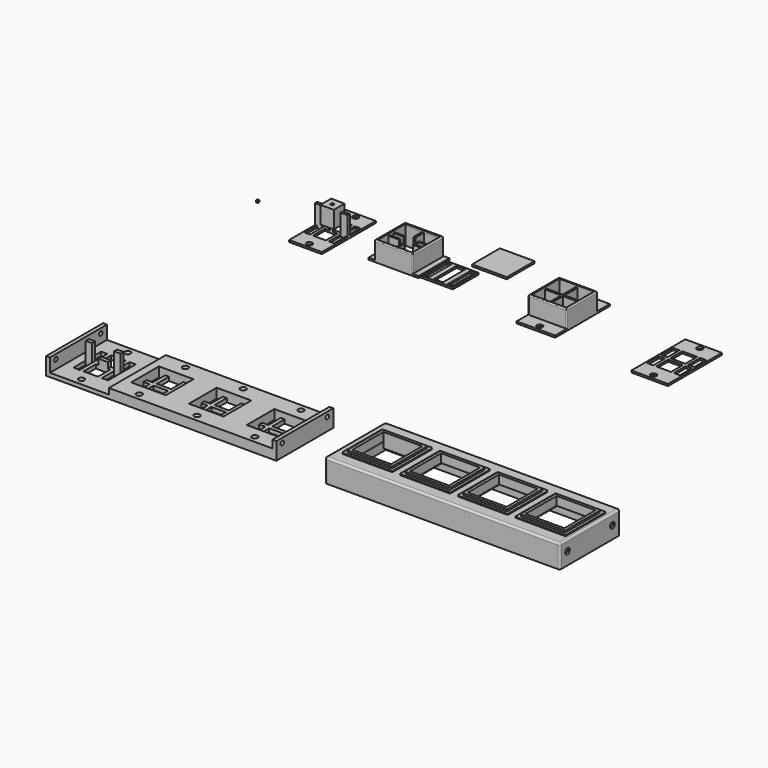
from build123d import *

# Parameters (mm, degrees)
F0_W          = 20
F0_H          = 20
F1_DEPTH      = 10
F2_T          = -1
F4_DEPTH      = 9
F5_W          = 20
F5_H          = 8
F5_R          = 1.5
F6_DEPTH      = 1
F7_W          = 19
F7_H          = 19
F7_H_2        = 8
F7_R          = 1.5
F8_DEPTH      = 1
F9_W          = 20
F9_H          = 20
F10_DEPTH     = 10
F11_W         = 3
F11_H         = 20
F11_W_2       = 20
F12_DEPTH     = 0.95
F13_T         = 1
F13_T3_DEPTH  = 22
F14_W         = 8.5
F14_H         = 0.9
F15_DEPTH     = 9
F17_DEPTH     = 9
F18_W         = 17
F18_H         = 8
F18_R         = 1.5
F18_H_2       = 19
F19_DEPTH     = 1
F20_W         = 1.5
F20_H         = 1.5
F21_DEPTH     = 3
F22_W         = 7
F22_H         = 7
F22_W_2       = 1.5
F22_H_2       = 1.5
F23_DEPTH     = 9
F24_W         = 1
F24_H         = 1
F25_DEPTH     = 1
F27_DEPTH     = 10
F28_W         = 0.9
F28_H         = 14.7
F28_W_2       = 2.5
F28_H_2       = 0.8
F28_H_3       = 6
F28_H_4       = 1.1
F29_DEPTH     = 1
F30_W         = 117
F30_H         = 37
F30_R         = 1.5
F31_DEPTH     = 1
F32_W         = 122
F32_H         = 39.2
F32_W_2       = 20.2
F32_H_2       = 20.2
F33_DEPTH     = 11
F34_W         = 120
F34_H         = 37.2
F35_DEPTH     = 8
F36_W         = 4
F36_H         = 18
F37_DEPTH     = 3
F39_W         = 3.25
F39_H         = 2
F40_DEPTH     = 9
F41_W         = 5
F41_H         = 2
F42_DEPTH     = 3
F43_R         = 1
F44_R         = 0.5
F44_2_R       = 0.5
F38_R         = 1.5
F45_DEPTH     = 3
F46_DEPTH     = 2
F47_W         = 2
F47_H         = 37
F48_DEPTH     = 7
F49_W         = 20.2
F49_H         = 8.5
F50_DEPTH     = 3
F51_R         = 1.5
F52_DEPTH     = 3
F54_R         = 1.5
F55_DEPTH     = 2
F56_W         = 3
F56_H         = 37.2
F57_DEPTH     = 1
F58_DEPTH     = 1
F59_W         = 2
F59_H         = 37
F60_DEPTH     = 4
F53_R         = 1.1
F61_DEPTH     = 269.2358512024
F62_DEPTH     = 3
F63_DEPTH     = 5
F46_FACE2_W   = 119
F46_FACE2_H   = 37
F46_FACE2_R   = 1.5
F46_FACE2_W_2 = 3.25
F46_FACE2_H_2 = 8
F46_FACE2_W_3 = 7.5
F64_DEPTH     = 1
F65_DEPTH     = 1
F66_DEPTH     = 2
F67_DEPTH     = 0.05
F69_W         = 20.2
F69_H         = 3
F70_DEPTH     = 0.5
F71_W         = 20.2
F71_H         = 1.5
F72_DEPTH     = 1
F73_R         = 0.5
F74_W         = 18
F74_H         = 17.9999990673
F75_DEPTH     = 1
F76_W         = 18
F76_H         = 18
F77_DEPTH     = 1
F78_W         = 18
F78_H         = 18
F79_DEPTH     = 1


# Not quite as in the source:
# - a shell that OpenCascade refuses in one call is made with other operations: the cavity is built on its own and cut out
# - a feature names something its author has since deleted; it is built from what else it names


with BuildPart() as f1:
    # F0 (on Top) → F1 (new body)
    with BuildSketch(Plane.XY):
        Rectangle(F0_W, F0_H)
    extrude(amount=F1_DEPTH)

    # F2
    f2_openings = [f1.faces().sort_by_distance(p)[0] for p in [
        (0, 0, 0),
    ]]
    offset(amount=F2_T, openings=f2_openings)

    # F3 (on Top) → F4 (join)
    with BuildSketch(Plane.XY):
        Polygon((-0.5, -9), (0.5, -9), (0.5, -0.5), (9, -0.5), (9, 0.5), (0.5, 0.5), (0.5, 9), (-0.5, 9), (-0.5, 0.5), (-9, 0.5), (-9, -0.5), (-0.5, -0.5), align=None)
    extrude(amount=F4_DEPTH)

    # F5 (on Top) → F6 (join)
    with BuildSketch(Plane.XY):
        with Locations((0, -13.5)):
            Rectangle(F5_W, F5_H)
        with Locations((0, -15)):
            Circle(F5_R, mode=Mode.SUBTRACT)
        with Locations((0, 14)):
            Rectangle(F5_W, F5_H)
        with Locations((0, 15)):
            Circle(F5_R, mode=Mode.SUBTRACT)
    extrude(amount=F6_DEPTH)

    # F44
    f44_edges = [f1.edges().sort_by_distance(p)[0] for p in [
        (-10, -10, 5.5),
        (0, -10, 10),
        (10, -10, 5.5),
        (-10, 0, 10),
        (-10, 10, 5.5),
        (0, 10, 10),
        (10, 10, 5.5),
        (10, 0, 10),
    ]]
    fillet(f44_edges, radius=F44_R)

    # F78 (on face) → F79 (cut)
    with BuildSketch(Plane.XY.offset(10)):
        Rectangle(F78_W, F78_H)
    extrude(amount=-F79_DEPTH, mode=Mode.SUBTRACT)


with BuildPart() as f8:
    # F7 (on Top) → F8 (new body)
    with BuildSketch(Plane.XY):
        with Locations((62.8032131791, -4.6075988114)):
            Rectangle(F7_W, F7_H)
        Polygon((54.3032131791, -3.8575988114), (54.3032131791, 3.8924011886), (57.4282131791, 3.8924011886), (58.9282131791, 3.8924011886), (66.6782131791, 3.8924011886), (68.1782131791, 3.8924011886), (71.3032131791, 3.8924011886), (71.3032131791, -3.8575988114), (71.3032131791, -5.3575988114), (71.3032131791, -13.1075988114), (68.1782131791, -13.1075988114), (66.6782131791, -13.1075988114), (58.9282131791, -13.1075988114), (57.4282131791, -13.1075988114), (54.3032131791, -13.1075988114), (54.3032131791, -5.3575988114), align=None, mode=Mode.SUBTRACT)
        with Locations((62.8032131791, 8.8924011886)):
            Rectangle(F7_W, F7_H_2)
        with Locations((62.8032131791, 10.3924011886)):
            Circle(F7_R, mode=Mode.SUBTRACT)
        with Locations((62.8032131791, -18.1075988114)):
            Rectangle(F7_W, F7_H_2)
        with Locations((62.8032131791, -19.6075988114)):
            Circle(F7_R, mode=Mode.SUBTRACT)
        Polygon((58.9282131791, 3.8924011886), (57.4282131791, 3.8924011886), (57.4282131791, -3.8575988114), (54.3032131791, -3.8575988114), (54.3032131791, -5.3575988114), (57.4282131791, -5.3575988114), (57.4282131791, -13.1075988114), (58.9282131791, -13.1075988114), (58.9282131791, -5.3575988114), (66.6782131791, -5.3575988114), (66.6782131791, -13.1075988114), (68.1782131791, -13.1075988114), (68.1782131791, -5.3575988114), (71.3032131791, -5.3575988114), (71.3032131791, -3.8575988114), (68.1782131791, -3.8575988114), (68.1782131791, 3.8924011886), (66.6782131791, 3.8924011886), (66.6782131791, -3.8575988114), (58.9282131791, -3.8575988114), align=None)
    extrude(amount=F8_DEPTH)


with BuildPart() as f10:
    # F9 (on Top) → F10 (new body)
    with BuildSketch(Plane.XY):
        with Locations((-78.8846665621, -1.3073290847)):
            Rectangle(F9_W, F9_H)
    extrude(amount=F10_DEPTH)

    # F11 (on face) → F12 (join)
    with BuildSketch(Plane(origin=(0, 0, 0), x_dir=(1, 0, 0), z_dir=(0, 0, -1))):
        with Locations((-90.3846665621, 1.3073290847)):
            Rectangle(F11_W, F11_H)
        with Locations((-78.8846665621, 1.3073290847)):
            Rectangle(F11_W_2, F11_H)
        with Locations((-67.3846665621, 1.3073290847)):
            Rectangle(F11_W, F11_H)
    extrude(amount=-F12_DEPTH)

    # F13: shell of thickness 1, made by hand


with BuildPart() as f13_core1:
    # F13_t2: copy of F10
    add(f10.part)

    # the walls: a layer under each face that stays
    f13_faces = [f13_core1.faces().sort_by_distance(p)[0] for p in [
        (-78.8846665621, 8.6926709153, 5),
        (-91.8846665621, -1.3073290847, 0.475),
        (-78.8846665621, -11.3073290847, 5),
        (-90.3846665621, -1.3073290847, 0.95),
        (-88.8846665621, -1.3073290847, 5.475),
        (-78.8846665621, -1.3073290847, 10),
        (-68.8846665621, -1.3073290847, 5.475),
        (-67.3846665621, -1.3073290847, 0.95),
        (-65.8846665621, -1.3073290847, 0.475),
    ]]
    thicken(f13_faces, amount=-F13_T, mode=Mode.SUBTRACT)

    # F13_s4 → F13_t3 (cut)
    with BuildSketch(Plane.XZ.offset(-9.6926709153)):
        Polygon((-88.8946665621, 0.96), (-88.8846665621, -0.05), (-87.8846665621, -0.05), (-87.8846665621, 0.95), align=None)
        Polygon((-68.8746665621, 0.96), (-69.8846665621, 0.95), (-69.8846665621, -0.05), (-68.8846665621, -0.05), align=None)
    extrude(amount=F13_T3_DEPTH, mode=Mode.SUBTRACT)


with BuildPart() as f10_1:
    add(f10.part)

    # what is left inside the walls is the cavity
    f13_cavity = [f13_core1.part.solids().sort_by_distance(p)[0] for p in [
        (-78.884667, -4.307329, 0.01),
    ]]
    add(f13_cavity, mode=Mode.SUBTRACT)

    # F14 (on Top) → F15 (join)
    with BuildSketch(Plane.XY):
        Polygon((-78.3846665621, 7.6926709153), (-79.3846665621, 7.6926709153), (-79.3846665621, 0.6926709153), (-79.3846665621, -0.2073290847), (-79.3846665621, -2.4073290847), (-79.3846665621, -3.3073290847), (-79.3846665621, -10.3073290847), (-78.3846665621, -10.3073290847), (-78.3846665621, -3.3073290847), (-78.3846665621, -2.4073290847), (-78.3846665621, -0.2073290847), (-78.3846665621, 0.6926709153), align=None)
        with Locations((-83.6346665621, -2.8573290847)):
            Rectangle(F14_W, F14_H)
        with Locations((-83.6346665621, 0.2426709153)):
            Rectangle(F14_W, F14_H)
        with Locations((-74.1346665621, 0.2426709153)):
            Rectangle(F14_W, F14_H)
        with Locations((-74.1346665621, -2.8573290847)):
            Rectangle(F14_W, F14_H)
    extrude(amount=F15_DEPTH)

    # F16 (on face) → F17 (cut)
    with BuildSketch(Plane(origin=(0, 0, 0), x_dir=(1, 0, 0), z_dir=(0, 0, -1))):
        Polygon((-79.3846665621, -2.2926709153), (-78.3846665621, -2.2926709153), (-78.3846665621, -0.6926709153), (-75.2846665621, -0.6926709153), (-75.2846665621, 0.2073290847), (-78.3846665621, 0.2073290847), (-78.3846665621, 2.4073290847), (-75.2846665621, 2.4073290847), (-75.2846665621, 3.3073290847), (-78.3846665621, 3.3073290847), (-78.3846665621, 4.9073290847), (-79.3846665621, 4.9073290847), (-79.3846665621, 3.3073290847), (-82.4846665621, 3.3073290847), (-82.4846665621, 2.4073290847), (-79.3846665621, 2.4073290847), (-79.3846665621, 0.2073290847), (-82.4846665621, 0.2073290847), (-82.4846665621, -0.6926709153), (-79.3846665621, -0.6926709153), align=None)
    extrude(amount=-F17_DEPTH, mode=Mode.SUBTRACT)

    # F44#2
    f44_2_edges = [f10_1.edges().sort_by_distance(p)[0] for p in [
        (-68.884667, -11.307329, 5.475),
        (-78.884667, -11.307329, 10),
        (-68.884667, -1.307329, 10),
        (-68.884667, 8.692671, 5.475),
        (-78.884667, 8.692671, 10),
        (-88.884667, 8.692671, 5.475),
        (-88.884667, -1.307329, 10),
        (-88.884667, -11.307329, 5.475),
    ]]
    fillet(f44_2_edges, radius=F44_2_R)

    # F67 (add): faces of the model
    f67_faces = [f10_1.faces().sort_by_distance(p)[0] for p in [
        (-90.3817894545, -1.3073290847, 0.95),
        (-67.3875436696, -1.3073290847, 0.95),
    ]]
    extrude(f67_faces, amount=F67_DEPTH)

    # F74 (on face) → F75 (cut)
    with BuildSketch(Plane.XY.offset(10)):
        with Locations((-78.8846665621, -1.3073295511)):
            Rectangle(F74_W, F74_H)
    extrude(amount=-F75_DEPTH, mode=Mode.SUBTRACT)


with BuildPart() as f19:
    # F18 (on Top) → F19 (new body)
    with BuildSketch(Plane.XY):
        with Locations((-118.1940851788, 11.6607970074)):
            Rectangle(F18_W, F18_H)
        with Locations((-118.1940851788, 13.1607970074)):
            Circle(F18_R, mode=Mode.SUBTRACT)
        with Locations((-118.1940851788, -15.3392029926)):
            Rectangle(F18_W, F18_H)
        with Locations((-118.1940851788, -16.8392029926)):
            Circle(F18_R, mode=Mode.SUBTRACT)
        with Locations((-118.1940851788, -1.8392029926)):
            Rectangle(F18_W, F18_H_2)
        Polygon((-125.6940851788, -1.0892029926), (-125.6940851788, 6.6607970074), (-123.0690851788, 6.6607970074), (-121.5690851788, 6.6607970074), (-114.8190851788, 6.6607970074), (-113.3190851788, 6.6607970074), (-110.6940851788, 6.6607970074), (-110.6940851788, -1.0892029926), (-110.6940851788, -2.5892029926), (-110.6940851788, -10.3392029926), (-113.3190851788, -10.3392029926), (-114.8190851788, -10.3392029926), (-121.5690851788, -10.3392029926), (-123.0690851788, -10.3392029926), (-125.6940851788, -10.3392029926), (-125.6940851788, -2.5892029926), align=None, mode=Mode.SUBTRACT)
        Polygon((-121.5690851788, 6.6607970074), (-123.0690851788, 6.6607970074), (-123.0690851788, -1.0892029926), (-125.6940851788, -1.0892029926), (-125.6940851788, -2.5892029926), (-123.0690851788, -2.5892029926), (-123.0690851788, -10.3392029926), (-121.5690851788, -10.3392029926), (-121.5690851788, -2.5892029926), (-114.8190851788, -2.5892029926), (-114.8190851788, -10.3392029926), (-113.3190851788, -10.3392029926), (-113.3190851788, -2.5892029926), (-110.6940851788, -2.5892029926), (-110.6940851788, -1.0892029926), (-113.3190851788, -1.0892029926), (-113.3190851788, 6.6607970074), (-114.8190851788, 6.6607970074), (-114.8190851788, -1.0892029926), (-121.5690851788, -1.0892029926), align=None)
    extrude(amount=F19_DEPTH)

    # F20 (on face) → F21 (join)
    with BuildSketch(Plane.XY.offset(1)):
        with Locations((-118.1940851788, -1.8392029926)):
            Rectangle(F20_W, F20_H)
    extrude(amount=F21_DEPTH)

    # F26 (on face) → F27 (join)
    with BuildSketch(Plane.XY.offset(1)):
        Polygon((-109.6940851788, -2.5892029926), (-109.6940851788, -1.0892029926), (-110.6940851788, -1.0892029926), (-113.3190851788, -1.0892029926), (-113.3190851788, -2.5892029926), (-110.6940851788, -2.5892029926), align=None)
        Polygon((-125.6940851788, -1.0892029926), (-126.6940851788, -1.0892029926), (-126.6940851788, -2.5892029926), (-125.6940851788, -2.5892029926), (-123.0690851788, -2.5892029926), (-123.0690851788, -1.0892029926), align=None)
    extrude(amount=F27_DEPTH)


with BuildPart() as f23:
    # F22 (on face) → F23 (new body)
    with BuildSketch(Plane.XY.offset(4)):
        with Locations((-118.1940851788, -1.8392029926)):
            Rectangle(F22_W, F22_H)
        with Locations((-118.1940851788, -1.8392029926)):
            Rectangle(F22_W_2, F22_H_2, mode=Mode.SUBTRACT)
    extrude(amount=F23_DEPTH)


with BuildPart() as f25:
    # F24 (on Top) → F25 (new body)
    with BuildSketch(Plane.XY):
        with Locations((-158.5527062416, 0)):
            Rectangle(F24_W, F24_H)
    extrude(amount=F25_DEPTH)


with BuildPart() as f29:
    # F28 (on Top) → F29 (new body)
    with BuildSketch(Plane.XY):
        Polygon((-64.4713718057, -9.4157041669), (-65.3713718057, -9.4157041669), (-65.3713718057, -10.3157041669), (-54.7713718057, -10.3157041669), (-52.2713718057, -10.3157041669), (-48.8713718057, -10.3157041669), (-48.8713718057, -9.4157041669), (-49.7713718057, -9.4157041669), (-52.2713718057, -9.4157041669), (-54.7713718057, -9.4157041669), (-59.4713718057, -9.4157041669), (-61.9713718057, -9.4157041669), align=None)
        with Locations((-64.9213718057, -2.0657041669)):
            Rectangle(F28_W, F28_H)
        Polygon((-48.8713718057, 6.1842958331), (-65.3713718057, 6.1842958331), (-65.3713718057, 5.2842958331), (-64.4713718057, 5.2842958331), (-61.9713718057, 5.2842958331), (-59.4713718057, 5.2842958331), (-54.7713718057, 5.2842958331), (-52.2713718057, 5.2842958331), (-49.7713718057, 5.2842958331), (-48.8713718057, 5.2842958331), align=None)
        with Locations((-49.3213718057, -2.0657041669)):
            Rectangle(F28_W, F28_H)
        with Locations((-53.5213718057, 4.8842958331)):
            Rectangle(F28_W_2, F28_H_2)
        with Locations((-53.5213718057, 1.4842958331)):
            Rectangle(F28_W_2, F28_H_3)
        with Locations((-53.5213718057, -2.0657041669)):
            Rectangle(F28_W_2, F28_H_4)
        with Locations((-53.5213718057, -5.6157041669)):
            Rectangle(F28_W_2, F28_H_3)
        with Locations((-53.5213718057, -9.0157041669)):
            Rectangle(F28_W_2, F28_H_2)
        with Locations((-60.7213718057, 4.8842958331)):
            Rectangle(F28_W_2, F28_H_2)
        with Locations((-60.7213718057, 1.4842958331)):
            Rectangle(F28_W_2, F28_H_3)
        with Locations((-60.7213718057, -2.0657041669)):
            Rectangle(F28_W_2, F28_H_4)
        with Locations((-60.7213718057, -5.6157041669)):
            Rectangle(F28_W_2, F28_H_3)
        with Locations((-60.7213718057, -9.0157041669)):
            Rectangle(F28_W_2, F28_H_2)
    extrude(amount=F29_DEPTH)


with BuildPart() as f31:
    # F30 (on Top) → F31 (new body)
    with BuildSketch(Plane.XY):
        with Locations((-71.0754835367, -152.5580135584)):
            Rectangle(F30_W, F30_H)
        with Locations((-115.9754835367, -167.5580135584)):
            Circle(F30_R, mode=Mode.SUBTRACT)
        with Locations((-85.9754835367, -167.5580135584)):
            Circle(F30_R, mode=Mode.SUBTRACT)
        Polygon((-124.9754835367, -151.5580135584), (-124.9754835367, -143.5580135584), (-121.7254835367, -143.5580135584), (-119.7254835367, -143.5580135584), (-112.2254835367, -143.5580135584), (-110.2254835367, -143.5580135584), (-106.9754835367, -143.5580135584), (-106.9754835367, -151.5580135584), (-106.9754835367, -153.5580135584), (-106.9754835367, -161.5580135584), (-110.2254835367, -161.5580135584), (-112.2254835367, -161.5580135584), (-119.7254835367, -161.5580135584), (-121.7254835367, -161.5580135584), (-124.9754835367, -161.5580135584), (-124.9754835367, -153.5580135584), align=None, mode=Mode.SUBTRACT)
        Polygon((-94.9754835367, -151.5580135584), (-94.9754835367, -143.5580135584), (-91.7254835367, -143.5580135584), (-89.7254835367, -143.5580135584), (-82.2254835367, -143.5580135584), (-80.2254835367, -143.5580135584), (-76.9754835367, -143.5580135584), (-76.9754835367, -151.5580135584), (-76.9754835367, -153.5580135584), (-76.9754835367, -161.5580135584), (-80.2254835367, -161.5580135584), (-82.2254835367, -161.5580135584), (-89.7254835367, -161.5580135584), (-91.7254835367, -161.5580135584), (-94.9754835367, -161.5580135584), (-94.9754835367, -153.5580135584), align=None, mode=Mode.SUBTRACT)
        with Locations((-55.9754835367, -167.5580135584)):
            Circle(F30_R, mode=Mode.SUBTRACT)
        with Locations((-25.9754835367, -167.5580135584)):
            Circle(F30_R, mode=Mode.SUBTRACT)
        Polygon((-64.9754835367, -151.5580135584), (-64.9754835367, -143.5580135584), (-61.7254835367, -143.5580135584), (-59.7254835367, -143.5580135584), (-52.2254835367, -143.5580135584), (-50.2254835367, -143.5580135584), (-46.9754835367, -143.5580135584), (-46.9754835367, -151.5580135584), (-46.9754835367, -153.5580135584), (-46.9754835367, -161.5580135584), (-47.9754835367, -161.5580135584), (-50.2254835367, -161.5580135584), (-52.2254835367, -161.5580135584), (-59.7254835367, -161.5580135584), (-61.7254835367, -161.5580135584), (-64.9754835367, -161.5580135584), (-64.9754835367, -153.5580135584), align=None, mode=Mode.SUBTRACT)
        Polygon((-34.9754835367, -151.5580135584), (-34.9754835367, -143.5580135584), (-31.7254835367, -143.5580135584), (-29.7254835367, -143.5580135584), (-22.2254835367, -143.5580135584), (-20.2254835367, -143.5580135584), (-16.9754835367, -143.5580135584), (-16.9754835367, -151.5580135584), (-16.9754835367, -153.5580135584), (-16.9754835367, -161.5580135584), (-17.9754835367, -161.5580135584), (-20.2254835367, -161.5580135584), (-22.2254835367, -161.5580135584), (-29.7254835367, -161.5580135584), (-31.7254835367, -161.5580135584), (-34.9754835367, -161.5580135584), (-34.9754835367, -153.5580135584), align=None, mode=Mode.SUBTRACT)
        with Locations((-115.9754835367, -137.5580135584)):
            Circle(F30_R, mode=Mode.SUBTRACT)
        with Locations((-85.9754835367, -137.5580135584)):
            Circle(F30_R, mode=Mode.SUBTRACT)
        with Locations((-55.9754835367, -137.5580135584)):
            Circle(F30_R, mode=Mode.SUBTRACT)
        with Locations((-25.9754835367, -137.5580135584)):
            Circle(F30_R, mode=Mode.SUBTRACT)
        Polygon((-119.7254835367, -143.5580135584), (-121.7254835367, -143.5580135584), (-121.7254835367, -151.5580135584), (-124.9754835367, -151.5580135584), (-124.9754835367, -153.5580135584), (-121.7254835367, -153.5580135584), (-121.7254835367, -161.5580135584), (-119.7254835367, -161.5580135584), (-119.7254835367, -153.5580135584), (-112.2254835367, -153.5580135584), (-112.2254835367, -161.5580135584), (-110.2254835367, -161.5580135584), (-110.2254835367, -153.5580135584), (-106.9754835367, -153.5580135584), (-106.9754835367, -151.5580135584), (-110.2254835367, -151.5580135584), (-110.2254835367, -143.5580135584), (-112.2254835367, -143.5580135584), (-112.2254835367, -151.5580135584), (-119.7254835367, -151.5580135584), align=None)
        Polygon((-89.7254835367, -143.5580135584), (-91.7254835367, -143.5580135584), (-91.7254835367, -151.5580135584), (-94.9754835367, -151.5580135584), (-94.9754835367, -153.5580135584), (-91.7254835367, -153.5580135584), (-91.7254835367, -161.5580135584), (-89.7254835367, -161.5580135584), (-89.7254835367, -153.5580135584), (-82.2254835367, -153.5580135584), (-82.2254835367, -161.5580135584), (-80.2254835367, -161.5580135584), (-80.2254835367, -153.5580135584), (-76.9754835367, -153.5580135584), (-76.9754835367, -151.5580135584), (-80.2254835367, -151.5580135584), (-80.2254835367, -143.5580135584), (-82.2254835367, -143.5580135584), (-82.2254835367, -151.5580135584), (-89.7254835367, -151.5580135584), align=None)
        Polygon((-59.7254835367, -143.5580135584), (-61.7254835367, -143.5580135584), (-61.7254835367, -151.5580135584), (-64.9754835367, -151.5580135584), (-64.9754835367, -153.5580135584), (-61.7254835367, -153.5580135584), (-61.7254835367, -161.5580135584), (-59.7254835367, -161.5580135584), (-59.7254835367, -153.5580135584), (-52.2254835367, -153.5580135584), (-52.2254835367, -161.5580135584), (-50.2254835367, -161.5580135584), (-50.2254835367, -153.5580135584), (-46.9754835367, -153.5580135584), (-46.9754835367, -151.5580135584), (-50.2254835367, -151.5580135584), (-50.2254835367, -143.5580135584), (-52.2254835367, -143.5580135584), (-52.2254835367, -151.5580135584), (-59.7254835367, -151.5580135584), align=None)
        Polygon((-29.7254835367, -143.5580135584), (-31.7254835367, -143.5580135584), (-31.7254835367, -151.5580135584), (-34.9754835367, -151.5580135584), (-34.9754835367, -153.5580135584), (-31.7254835367, -153.5580135584), (-31.7254835367, -161.5580135584), (-29.7254835367, -161.5580135584), (-29.7254835367, -153.5580135584), (-22.2254835367, -153.5580135584), (-22.2254835367, -161.5580135584), (-20.2254835367, -161.5580135584), (-20.2254835367, -153.5580135584), (-16.9754835367, -153.5580135584), (-16.9754835367, -151.5580135584), (-20.2254835367, -151.5580135584), (-20.2254835367, -143.5580135584), (-22.2254835367, -143.5580135584), (-22.2254835367, -151.5580135584), (-29.7254835367, -151.5580135584), align=None)
    extrude(amount=F31_DEPTH)

    # F36 (on face) → F37 (join)
    with BuildSketch(Plane.XY.offset(1)):
        with Locations((-96.9754835367, -152.5580135584)):
            Rectangle(F36_W, F36_H)
        with Locations((-74.9754835367, -152.5580135584)):
            Rectangle(F36_W, F36_H)
        with Locations((-66.9754835367, -152.5580135584)):
            Rectangle(F36_W, F36_H)
        with Locations((-44.9754835367, -152.5580135584)):
            Rectangle(F36_W, F36_H)
        with Locations((-36.9754835367, -152.5580135584)):
            Rectangle(F36_W, F36_H)
        with Locations((-14.9754835367, -152.5580135584)):
            Rectangle(F36_W, F36_H)
    extrude(amount=F37_DEPTH)

    # F39 (on face) → F40 (join)
    with BuildSketch(Plane.XY.offset(1)):
        with Locations((-123.3504835367, -152.5580135584)):
            Rectangle(F39_W, F39_H)
        with Locations((-108.6004835367, -152.5580135584)):
            Rectangle(F39_W, F39_H)
    extrude(amount=F40_DEPTH)

    # F41 (on face) → F42 (join)
    with BuildSketch(Plane.XY.offset(1)):
        with Locations((-115.9754835367, -152.5580135584)):
            Rectangle(F41_W, F41_H)
    extrude(amount=F42_DEPTH)

    # F38 (on face) → F45 (join)
    with BuildSketch(Plane.XY.offset(1)):
        Polygon((-98.9754835367, -134.0580135584), (-98.9754835367, -143.5580135584), (-94.9754835367, -143.5580135584), (-91.7254835367, -143.5580135584), (-89.7254835367, -143.5580135584), (-82.2254835367, -143.5580135584), (-80.2254835367, -143.5580135584), (-76.9754835367, -143.5580135584), (-72.9754835367, -143.5580135584), (-72.9754835367, -134.0580135584), align=None)
        with Locations((-85.9754835367, -137.5580135584)):
            Circle(F38_R, mode=Mode.SUBTRACT)
        Polygon((-94.9754835367, -161.5580135584), (-98.9754835367, -161.5580135584), (-98.9754835367, -171.0580135584), (-72.9754835367, -171.0580135584), (-72.9754835367, -161.5580135584), (-76.9754835367, -161.5580135584), (-80.2254835367, -161.5580135584), (-82.2254835367, -161.5580135584), (-89.7254835367, -161.5580135584), (-91.7254835367, -161.5580135584), align=None)
        with Locations((-85.9754835367, -167.5580135584)):
            Circle(F38_R, mode=Mode.SUBTRACT)
        Polygon((-68.9754835367, -161.5580135584), (-68.9754835367, -171.0580135584), (-42.9754835367, -171.0580135584), (-42.9754835367, -161.5580135584), (-46.9754835367, -161.5580135584), (-50.2254835367, -161.5580135584), (-52.2254835367, -161.5580135584), (-59.7254835367, -161.5580135584), (-61.7254835367, -161.5580135584), (-64.9754835367, -161.5580135584), align=None)
        with Locations((-55.9754835367, -167.5580135584)):
            Circle(F38_R, mode=Mode.SUBTRACT)
        Polygon((-42.9754835367, -134.0580135584), (-68.9754835367, -134.0580135584), (-68.9754835367, -143.5580135584), (-64.9754835367, -143.5580135584), (-61.7254835367, -143.5580135584), (-59.7254835367, -143.5580135584), (-52.2254835367, -143.5580135584), (-50.2254835367, -143.5580135584), (-46.9754835367, -143.5580135584), (-42.9754835367, -143.5580135584), align=None)
        with Locations((-55.9754835367, -137.5580135584)):
            Circle(F38_R, mode=Mode.SUBTRACT)
        Polygon((-12.9754835367, -134.0580135584), (-38.9754835367, -134.0580135584), (-38.9754835367, -143.5580135584), (-34.9754835367, -143.5580135584), (-31.7254835367, -143.5580135584), (-29.7254835367, -143.5580135584), (-22.2254835367, -143.5580135584), (-20.2254835367, -143.5580135584), (-16.9754835367, -143.5580135584), (-12.9754835367, -143.5580135584), align=None)
        with Locations((-25.9754835367, -137.5580135584)):
            Circle(F38_R, mode=Mode.SUBTRACT)
        Polygon((-38.9754835367, -161.5580135584), (-38.9754835367, -171.0580135584), (-12.9754835367, -171.0580135584), (-12.9754835367, -161.5580135584), (-16.9754835367, -161.5580135584), (-20.2254835367, -161.5580135584), (-22.2254835367, -161.5580135584), (-29.7254835367, -161.5580135584), (-31.7254835367, -161.5580135584), (-34.9754835367, -161.5580135584), align=None)
        with Locations((-25.9754835367, -167.5580135584)):
            Circle(F38_R, mode=Mode.SUBTRACT)
    extrude(amount=F45_DEPTH)

    # F46 (add): a face of the model
    f46_faces = [f31.faces().sort_by_distance(p)[0] for p in [
        (-129.5754835367, -152.5580135584, 0.5),
    ]]
    extrude(f46_faces, amount=F46_DEPTH)

    # F47 (on face) → F48 (join)
    with BuildSketch(Plane.XY.offset(1)):
        with Locations((-130.5754835367, -152.5580135584)):
            Rectangle(F47_W, F47_H)
    extrude(amount=F48_DEPTH)

    # F58 (add): a face of the model
    f58_faces = [f31.faces().sort_by_distance(p)[0] for p in [
        (-12.9754835367, -152.5580135584, 2.5),
    ]]
    extrude(f58_faces, amount=F58_DEPTH)

    # F59 (on face) → F60 (join)
    with BuildSketch(Plane.XY.offset(4)):
        with Locations((-12.9754835367, -152.5580135584)):
            Rectangle(F59_W, F59_H)
    extrude(amount=F60_DEPTH)

    # F53 (on face) → F61 (cut, through all)
    with BuildSketch(Plane(origin=(-131.5754835367, 0, 0), x_dir=(0, -1, 0), z_dir=(-1, 0, 0))):
        with Locations((137.9580135584, 5.5)):
            Circle(F53_R)
        with Locations((167.1580135584, 5.5)):
            Circle(F53_R)
    extrude(amount=-F61_DEPTH, mode=Mode.SUBTRACT)

    # F63 (add): faces of the model
    f63_faces = [f31.faces().sort_by_distance(p)[0] for p in [
        (-72.9754835367, -152.5580135584, 2.5),
        (-42.9754835367, -152.5580135584, 2.5),
    ]]
    extrude(f63_faces, amount=F63_DEPTH)

    # F30 (on Top) + F46_face2 (on face) → F64 (join)
    with BuildSketch(Plane.XY):
        with Locations((-71.0754835367, -152.5580135584)):
            Rectangle(F30_W, F30_H)
        with Locations((-115.9754835367, -167.5580135584)):
            Circle(F30_R, mode=Mode.SUBTRACT)
        with Locations((-85.9754835367, -167.5580135584)):
            Circle(F30_R, mode=Mode.SUBTRACT)
        Polygon((-124.9754835367, -151.5580135584), (-124.9754835367, -143.5580135584), (-121.7254835367, -143.5580135584), (-119.7254835367, -143.5580135584), (-112.2254835367, -143.5580135584), (-110.2254835367, -143.5580135584), (-106.9754835367, -143.5580135584), (-106.9754835367, -151.5580135584), (-106.9754835367, -153.5580135584), (-106.9754835367, -161.5580135584), (-110.2254835367, -161.5580135584), (-112.2254835367, -161.5580135584), (-119.7254835367, -161.5580135584), (-121.7254835367, -161.5580135584), (-124.9754835367, -161.5580135584), (-124.9754835367, -153.5580135584), align=None, mode=Mode.SUBTRACT)
        Polygon((-94.9754835367, -151.5580135584), (-94.9754835367, -143.5580135584), (-91.7254835367, -143.5580135584), (-89.7254835367, -143.5580135584), (-82.2254835367, -143.5580135584), (-80.2254835367, -143.5580135584), (-76.9754835367, -143.5580135584), (-76.9754835367, -151.5580135584), (-76.9754835367, -153.5580135584), (-76.9754835367, -161.5580135584), (-80.2254835367, -161.5580135584), (-82.2254835367, -161.5580135584), (-89.7254835367, -161.5580135584), (-91.7254835367, -161.5580135584), (-94.9754835367, -161.5580135584), (-94.9754835367, -153.5580135584), align=None, mode=Mode.SUBTRACT)
        with Locations((-55.9754835367, -167.5580135584)):
            Circle(F30_R, mode=Mode.SUBTRACT)
        with Locations((-25.9754835367, -167.5580135584)):
            Circle(F30_R, mode=Mode.SUBTRACT)
        Polygon((-64.9754835367, -151.5580135584), (-64.9754835367, -143.5580135584), (-61.7254835367, -143.5580135584), (-59.7254835367, -143.5580135584), (-52.2254835367, -143.5580135584), (-50.2254835367, -143.5580135584), (-46.9754835367, -143.5580135584), (-46.9754835367, -151.5580135584), (-46.9754835367, -153.5580135584), (-46.9754835367, -161.5580135584), (-47.9754835367, -161.5580135584), (-50.2254835367, -161.5580135584), (-52.2254835367, -161.5580135584), (-59.7254835367, -161.5580135584), (-61.7254835367, -161.5580135584), (-64.9754835367, -161.5580135584), (-64.9754835367, -153.5580135584), align=None, mode=Mode.SUBTRACT)
        Polygon((-34.9754835367, -151.5580135584), (-34.9754835367, -143.5580135584), (-31.7254835367, -143.5580135584), (-29.7254835367, -143.5580135584), (-22.2254835367, -143.5580135584), (-20.2254835367, -143.5580135584), (-16.9754835367, -143.5580135584), (-16.9754835367, -151.5580135584), (-16.9754835367, -153.5580135584), (-16.9754835367, -161.5580135584), (-17.9754835367, -161.5580135584), (-20.2254835367, -161.5580135584), (-22.2254835367, -161.5580135584), (-29.7254835367, -161.5580135584), (-31.7254835367, -161.5580135584), (-34.9754835367, -161.5580135584), (-34.9754835367, -153.5580135584), align=None, mode=Mode.SUBTRACT)
        with Locations((-115.9754835367, -137.5580135584)):
            Circle(F30_R, mode=Mode.SUBTRACT)
        with Locations((-85.9754835367, -137.5580135584)):
            Circle(F30_R, mode=Mode.SUBTRACT)
        with Locations((-55.9754835367, -137.5580135584)):
            Circle(F30_R, mode=Mode.SUBTRACT)
        with Locations((-25.9754835367, -137.5580135584)):
            Circle(F30_R, mode=Mode.SUBTRACT)
    with BuildSketch(Plane(origin=(-72.3791549796, -152.5580135584, 0), x_dir=(1, 0, 0), z_dir=(0, 0, -1))):
        with Locations((0.3036714428, 0)):
            Rectangle(F46_FACE2_W, F46_FACE2_H)
        with Locations((-43.5963285572, 15)):
            Circle(F46_FACE2_R, mode=Mode.SUBTRACT)
        with Locations((-13.5963285572, 15)):
            Circle(F46_FACE2_R, mode=Mode.SUBTRACT)
        with Locations((-36.2213285572, 5)):
            Rectangle(F46_FACE2_W_2, F46_FACE2_H_2, mode=Mode.SUBTRACT)
        with Locations((-43.5963285572, 5)):
            Rectangle(F46_FACE2_W_3, F46_FACE2_H_2, mode=Mode.SUBTRACT)
        with Locations((-50.9713285572, 5)):
            Rectangle(F46_FACE2_W_2, F46_FACE2_H_2, mode=Mode.SUBTRACT)
        with Locations((-50.9713285572, -5)):
            Rectangle(F46_FACE2_W_2, F46_FACE2_H_2, mode=Mode.SUBTRACT)
        with Locations((-43.5963285572, -5)):
            Rectangle(F46_FACE2_W_3, F46_FACE2_H_2, mode=Mode.SUBTRACT)
        with Locations((-36.2213285572, -5)):
            Rectangle(F46_FACE2_W_2, F46_FACE2_H_2, mode=Mode.SUBTRACT)
        with Locations((-6.2213285572, 5)):
            Rectangle(F46_FACE2_W_2, F46_FACE2_H_2, mode=Mode.SUBTRACT)
        with Locations((-13.5963285572, 5)):
            Rectangle(F46_FACE2_W_3, F46_FACE2_H_2, mode=Mode.SUBTRACT)
        with Locations((-20.9713285572, 5)):
            Rectangle(F46_FACE2_W_2, F46_FACE2_H_2, mode=Mode.SUBTRACT)
        with Locations((-20.9713285572, -5)):
            Rectangle(F46_FACE2_W_2, F46_FACE2_H_2, mode=Mode.SUBTRACT)
        with Locations((-13.5963285572, -5)):
            Rectangle(F46_FACE2_W_3, F46_FACE2_H_2, mode=Mode.SUBTRACT)
        with Locations((-6.2213285572, -5)):
            Rectangle(F46_FACE2_W_2, F46_FACE2_H_2, mode=Mode.SUBTRACT)
        with Locations((16.4036714428, 15)):
            Circle(F46_FACE2_R, mode=Mode.SUBTRACT)
        with Locations((46.4036714428, 15)):
            Circle(F46_FACE2_R, mode=Mode.SUBTRACT)
        with Locations((23.7786714428, 5)):
            Rectangle(F46_FACE2_W_2, F46_FACE2_H_2, mode=Mode.SUBTRACT)
        with Locations((16.4036714428, 5)):
            Rectangle(F46_FACE2_W_3, F46_FACE2_H_2, mode=Mode.SUBTRACT)
        with Locations((9.0286714428, 5)):
            Rectangle(F46_FACE2_W_2, F46_FACE2_H_2, mode=Mode.SUBTRACT)
        with Locations((9.0286714428, -5)):
            Rectangle(F46_FACE2_W_2, F46_FACE2_H_2, mode=Mode.SUBTRACT)
        with Locations((16.4036714428, -5)):
            Rectangle(F46_FACE2_W_3, F46_FACE2_H_2, mode=Mode.SUBTRACT)
        with Locations((23.7786714428, -5)):
            Rectangle(F46_FACE2_W_2, F46_FACE2_H_2, mode=Mode.SUBTRACT)
        with Locations((53.7786714428, 5)):
            Rectangle(F46_FACE2_W_2, F46_FACE2_H_2, mode=Mode.SUBTRACT)
        with Locations((46.4036714428, 5)):
            Rectangle(F46_FACE2_W_3, F46_FACE2_H_2, mode=Mode.SUBTRACT)
        with Locations((39.0286714428, 5)):
            Rectangle(F46_FACE2_W_2, F46_FACE2_H_2, mode=Mode.SUBTRACT)
        with Locations((39.0286714428, -5)):
            Rectangle(F46_FACE2_W_2, F46_FACE2_H_2, mode=Mode.SUBTRACT)
        with Locations((46.4036714428, -5)):
            Rectangle(F46_FACE2_W_3, F46_FACE2_H_2, mode=Mode.SUBTRACT)
        with Locations((53.7786714428, -5)):
            Rectangle(F46_FACE2_W_2, F46_FACE2_H_2, mode=Mode.SUBTRACT)
        with Locations((-43.5963285572, -15)):
            Circle(F46_FACE2_R, mode=Mode.SUBTRACT)
        with Locations((-13.5963285572, -15)):
            Circle(F46_FACE2_R, mode=Mode.SUBTRACT)
        with Locations((16.4036714428, -15)):
            Circle(F46_FACE2_R, mode=Mode.SUBTRACT)
        with Locations((46.4036714428, -15)):
            Circle(F46_FACE2_R, mode=Mode.SUBTRACT)
    extrude(amount=-F64_DEPTH, dir=(0, 0, 1))

    # F66 (add): a face of the model
    f66_faces = [f31.faces().sort_by_distance(p)[0] for p in [
        (-12.2754835367, -152.5580135584, 1),
    ]]
    extrude(f66_faces, amount=F66_DEPTH)


with BuildPart() as f33:
    # F32 (on Top) → F33 (new body)
    with BuildSketch(Plane.XY):
        with Locations((76.6593676656, -154.4580135584)):
            Rectangle(F32_W, F32_H)
        with Locations((32.3593676656, -154.4580135584)):
            Rectangle(F32_W_2, F32_H_2, mode=Mode.SUBTRACT)
        with Locations((62.3593676656, -154.4580135584)):
            Rectangle(F32_W_2, F32_H_2, mode=Mode.SUBTRACT)
        with Locations((92.3593676656, -154.4580135584)):
            Rectangle(F32_W_2, F32_H_2, mode=Mode.SUBTRACT)
        with Locations((122.3593676656, -154.4580135584)):
            Rectangle(F32_W_2, F32_H_2, mode=Mode.SUBTRACT)
    extrude(amount=F33_DEPTH)

    # F34 (on face) → F35 (cut)
    with BuildSketch(Plane(origin=(0, 0, 0), x_dir=(1, 0, 0), z_dir=(0, 0, -1))):
        with Locations((76.6593676656, 154.4580135584)):
            Rectangle(F34_W, F34_H)
    extrude(amount=-F35_DEPTH, mode=Mode.SUBTRACT)

    # F43
    f43_edges = [f33.edges().sort_by_distance(p)[0] for p in [
        (15.659368, -134.858014, 5.5),
        (15.659368, -174.058014, 5.5),
        (137.659368, -174.058014, 5.5),
        (137.659368, -134.858014, 5.5),
        (76.659368, -174.058014, 11),
        (15.659368, -154.458014, 11),
        (76.659368, -134.858014, 11),
        (137.659368, -154.458014, 11),
    ]]
    fillet(f43_edges, radius=F43_R)

    # F49 (on face) → F50 (join)
    with BuildSketch(Plane(origin=(0, 0, 8), x_dir=(1, 0, 0), z_dir=(0, 0, -1))):
        with Locations((32.3593676656, 168.8080135584)):
            Rectangle(F49_W, F49_H)
        with Locations((32.3593676656, 140.1080135584)):
            Rectangle(F49_W, F49_H)
    extrude(amount=F50_DEPTH)

    # F51 (on face) → F52 (cut)
    with BuildSketch(Plane(origin=(15.6593676656, 0, 0), x_dir=(0, -1, 0), z_dir=(-1, 0, 0))):
        with Locations((139.8580135584, 5.5)):
            Circle(F51_R)
        with Locations((169.0580135584, 5.5)):
            Circle(F51_R)
    extrude(amount=-F52_DEPTH, mode=Mode.SUBTRACT)

    # F54 (on face) → F55 (cut)
    with BuildSketch(Plane.YZ.offset(137.6593676656)):
        with Locations((-169.0580135584, 5.5)):
            Circle(F54_R)
        with Locations((-139.8580135584, 5.5)):
            Circle(F54_R)
    extrude(amount=-F55_DEPTH, mode=Mode.SUBTRACT)

    # F56 (on face) → F57 (join)
    with BuildSketch(Plane(origin=(0, 0, 8), x_dir=(1, 0, 0), z_dir=(0, 0, -1))):
        with Locations((47.4593676656, 154.4580135584)):
            Rectangle(F56_W, F56_H)
        with Locations((77.4593676656, 154.4580135584)):
            Rectangle(F56_W, F56_H)
        with Locations((107.4593676656, 154.4580135584)):
            Rectangle(F56_W, F56_H)
    extrude(amount=F57_DEPTH)

    # F56 (on face) → F62 (join)
    with BuildSketch(Plane(origin=(0, 0, 8), x_dir=(1, 0, 0), z_dir=(0, 0, -1))):
        with Locations((47.4593676656, 154.4580135584)):
            Rectangle(F56_W, F56_H)
        with Locations((77.4593676656, 154.4580135584)):
            Rectangle(F56_W, F56_H)
        with Locations((107.4593676656, 154.4580135584)):
            Rectangle(F56_W, F56_H)
    extrude(amount=F62_DEPTH)

    # F65 (add): a face of the model
    f65_faces = [f33.faces().sort_by_distance(p)[0] for p in [
        (137.5312246206, -154.4580135584, 0),
    ]]
    extrude(f65_faces, amount=F65_DEPTH)

    # F69 (on face) → F70 (join)
    with BuildSketch(Plane.XY.offset(11)):
        with Locations((32.3593676656, -142.8580135584)):
            Rectangle(F69_W, F69_H)
        Polygon((22.2593676656, -164.5580135584), (22.2593676656, -144.3580135584), (22.2593676656, -141.3580135584), (19.2593676656, -141.3580135584), (19.2593676656, -167.5580135584), (22.2593676656, -167.5580135584), align=None)
        Polygon((42.4593676656, -141.3580135584), (42.4593676656, -144.3580135584), (42.4593676656, -164.5580135584), (42.4593676656, -167.5580135584), (45.4593676656, -167.5580135584), (45.4593676656, -141.3580135584), align=None)
        with Locations((32.3593676656, -166.0580135584)):
            Rectangle(F69_W, F69_H)
        with Locations((62.3593676656, -142.8580135584)):
            Rectangle(F69_W, F69_H)
        Polygon((52.2593676656, -164.5580135584), (52.2593676656, -144.3580135584), (52.2593676656, -141.3580135584), (49.2593676656, -141.3580135584), (49.2593676656, -167.5580135584), (52.2593676656, -167.5580135584), align=None)
        Polygon((72.4593676656, -141.3580135584), (72.4593676656, -144.3580135584), (72.4593676656, -164.5580135584), (72.4593676656, -167.5580135584), (75.4593676656, -167.5580135584), (75.4593676656, -141.3580135584), align=None)
        with Locations((62.3593676656, -166.0580135584)):
            Rectangle(F69_W, F69_H)
        with Locations((92.3593676656, -142.8580135584)):
            Rectangle(F69_W, F69_H)
        Polygon((82.2593676656, -164.5580135584), (82.2593676656, -144.3580135584), (82.2593676656, -141.3580135584), (79.2593676656, -141.3580135584), (79.2593676656, -167.5580135584), (82.2593676656, -167.5580135584), align=None)
        Polygon((102.4593676656, -141.3580135584), (102.4593676656, -144.3580135584), (102.4593676656, -164.5580135584), (102.4593676656, -167.5580135584), (105.4593676656, -167.5580135584), (105.4593676656, -141.3580135584), align=None)
        with Locations((92.3593676656, -166.0580135584)):
            Rectangle(F69_W, F69_H)
        with Locations((122.3593676656, -142.8580135584)):
            Rectangle(F69_W, F69_H)
        Polygon((112.2593676656, -164.5580135584), (112.2593676656, -144.3580135584), (112.2593676656, -141.3580135584), (109.2593676656, -141.3580135584), (109.2593676656, -167.5580135584), (112.2593676656, -167.5580135584), align=None)
        Polygon((132.4593676656, -141.3580135584), (132.4593676656, -144.3580135584), (132.4593676656, -164.5580135584), (132.4593676656, -167.5580135584), (135.4593676656, -167.5580135584), (135.4593676656, -141.3580135584), align=None)
        with Locations((122.3593676656, -166.0580135584)):
            Rectangle(F69_W, F69_H)
    extrude(amount=F70_DEPTH)

    # F71 (on face) → F72 (join)
    with BuildSketch(Plane.XY.offset(11.5)):
        with Locations((32.3593676656, -143.6080135584)):
            Rectangle(F71_W, F71_H)
        Polygon((22.2593676656, -164.5580135584), (22.2593676656, -144.3580135584), (22.2593676656, -142.8580135584), (20.7593676656, -142.8580135584), (20.7593676656, -166.0580135584), (22.2593676656, -166.0580135584), align=None)
        Polygon((42.4593676656, -142.8580135584), (42.4593676656, -144.3580135584), (42.4593676656, -164.5580135584), (42.4593676656, -166.0580135584), (43.9593676656, -166.0580135584), (43.9593676656, -142.8580135584), align=None)
        with Locations((32.3593676656, -165.3080135584)):
            Rectangle(F71_W, F71_H)
        Polygon((52.2593676656, -142.8580135584), (50.7593676656, -142.8580135584), (50.7593676656, -166.0580135584), (52.2593676656, -166.0580135584), (52.2593676656, -164.5580135584), (52.2593676656, -144.3580135584), align=None)
        with Locations((62.3593676656, -143.6080135584)):
            Rectangle(F71_W, F71_H)
        Polygon((73.9593676656, -142.8580135584), (72.4593676656, -142.8580135584), (72.4593676656, -144.3580135584), (72.4593676656, -164.5580135584), (72.4593676656, -166.0580135584), (73.9593676656, -166.0580135584), align=None)
        with Locations((62.3593676656, -165.3080135584)):
            Rectangle(F71_W, F71_H)
        Polygon((82.2593676656, -142.8580135584), (80.7593676656, -142.8580135584), (80.7593676656, -166.0580135584), (82.2593676656, -166.0580135584), (82.2593676656, -164.5580135584), (82.2593676656, -144.3580135584), align=None)
        with Locations((92.3593676656, -143.6080135584)):
            Rectangle(F71_W, F71_H)
        Polygon((103.9593676656, -142.8580135584), (102.4593676656, -142.8580135584), (102.4593676656, -144.3580135584), (102.4593676656, -164.5580135584), (102.4593676656, -166.0580135584), (103.9593676656, -166.0580135584), align=None)
        with Locations((92.3593676656, -165.3080135584)):
            Rectangle(F71_W, F71_H)
        Polygon((112.2593676656, -142.8580135584), (110.7593676656, -142.8580135584), (110.7593676656, -166.0580135584), (112.2593676656, -166.0580135584), (112.2593676656, -164.5580135584), (112.2593676656, -144.3580135584), align=None)
        with Locations((122.3593676656, -143.6080135584)):
            Rectangle(F71_W, F71_H)
        Polygon((133.9593676656, -142.8580135584), (132.4593676656, -142.8580135584), (132.4593676656, -144.3580135584), (132.4593676656, -164.5580135584), (132.4593676656, -166.0580135584), (133.9593676656, -166.0580135584), align=None)
        with Locations((122.3593676656, -165.3080135584)):
            Rectangle(F71_W, F71_H)
    extrude(amount=F72_DEPTH)

    # F73
    f73_edges = [f33.edges().sort_by_distance(p)[0] for p in [
        (19.259368, -141.358014, 11.25),
        (20.759368, -142.858014, 12),
        (19.259368, -167.558014, 11.25),
        (20.759368, -166.058014, 12),
        (43.959368, -166.058014, 12),
        (45.459368, -167.558014, 11.25),
        (43.959368, -142.858014, 12),
        (45.459368, -141.358014, 11.25),
        (49.259368, -141.358014, 11.25),
        (50.759368, -142.858014, 12),
        (50.759368, -166.058014, 12),
        (49.259368, -167.558014, 11.25),
        (73.959368, -166.058014, 12),
        (75.459368, -167.558014, 11.25),
        (73.959368, -142.858014, 12),
        (75.459368, -141.358014, 11.25),
        (79.259368, -141.358014, 11.25),
        (80.759368, -142.858014, 12),
        (79.259368, -167.558014, 11.25),
        (80.759368, -166.058014, 12),
        (103.959368, -166.058014, 12),
        (105.459368, -167.558014, 11.25),
        (103.959368, -142.858014, 12),
        (105.459368, -141.358014, 11.25),
        (109.259368, -141.358014, 11.25),
        (110.759368, -142.858014, 12),
        (109.259368, -167.558014, 11.25),
        (110.759368, -166.058014, 12),
        (133.959368, -166.058014, 12),
        (135.459368, -167.558014, 11.25),
        (133.959368, -142.858014, 12),
        (135.459368, -141.358014, 11.25),
    ]]
    fillet(f73_edges, radius=F73_R)


with BuildPart() as f77:
    # F76 (on Top) → F77 (new body)
    with BuildSketch(Plane.XY):
        with Locations((-46.3569205403, 19.2935256436)):
            Rectangle(F76_W, F76_H)
    extrude(amount=F77_DEPTH)


solid = Compound([f1.part, f8.part, f10_1.part, f19.part, f23.part, f25.part, f29.part, f31.part, f33.part, f77.part])
